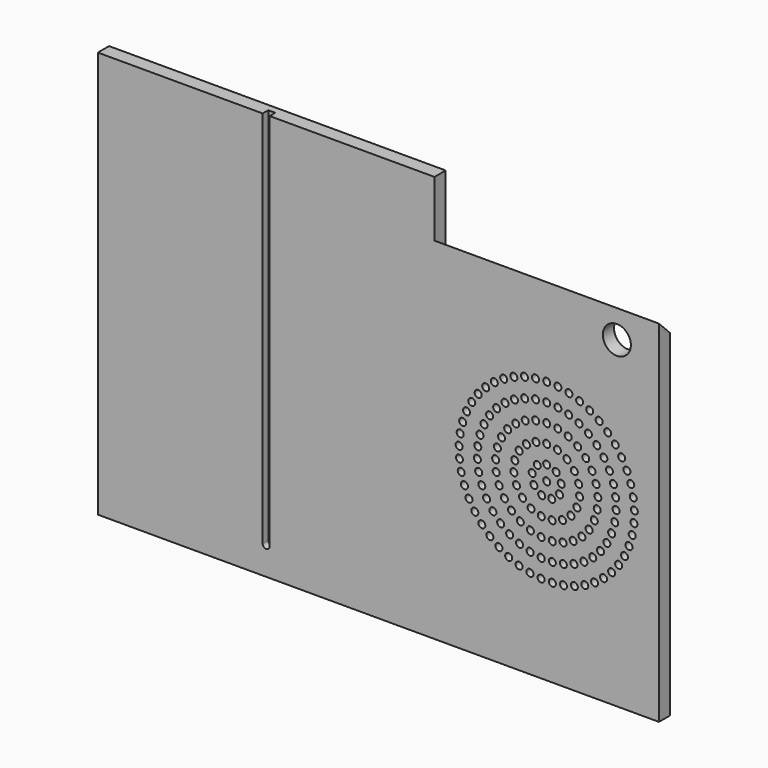
from build123d import *

# Parameters (mm, degrees)
F0_W     = 80
F0_H     = 125
F0_R     = 35
F0_R_2   = 5
F0_R_3   = 1.25
F1_DEPTH = 5
F2_DEPTH = 2.5
F3_SIZE2 = 4.99999
F3_SIZE  = 4.99999


# Not quite as in the source:
# - a fillet or chamfer is up to 0.001 mm smaller than in the source, because OpenCascade refuses the exact size


with BuildPart() as f1:
    # F0 (on Front) → F1 (new body)
    with BuildSketch(Plane.XZ):
        with BuildLine():
            Line((-78.9264041185, -49.894323349), (-78.9264041185, 75.105676651))
            Line((-78.9264041185, 75.105676651), (-78.9264041185, 95.105676651))
            Line((-78.9264041185, 95.105676651), (-137.6764041185, 95.105676651))
            Line((-137.6764041185, 95.105676651), (-137.6764041185, -39.8327037927))
            ThreePointArc((-137.6764041185, -39.8327037927), (-138.8948255892, -41.1447029883), (-140.1764041185, -39.894323349))
            Line((-140.1764041185, -39.894323349), (-140.1764041185, 95.105676651))
            Line((-140.1764041185, 95.105676651), (-198.9264041185, 95.105676651))
            Line((-198.9264041185, 95.105676651), (-198.9264041185, -49.894323349))
            Line((-198.9264041185, -49.894323349), (-78.9264041185, -49.894323349))
        make_face()
        with Locations((-38.9264041185, 12.605676651)):
            Rectangle(F0_W, F0_H)
        with Locations((-38.9264041185, 12.605676651)):
            Circle(F0_R, mode=Mode.SUBTRACT)
        with Locations((-13.9264041185, 65.105676651)):
            Circle(F0_R_2, mode=Mode.SUBTRACT)
        with Locations((-38.9264041185, 12.605676651)):
            Circle(F0_R)
        with Locations((-52.485270966, -15.5496004709)):
            Circle(F0_R_3, mode=Mode.SUBTRACT)
        with Locations((-40.9285984929, -18.5801168724)):
            Circle(F0_R_3, mode=Mode.SUBTRACT)
        with Locations((-36.9242097441, -18.5801168724)):
            Circle(F0_R_3, mode=Mode.SUBTRACT)
        with Locations((-48.7735359318, -17.0523154431)):
            Circle(F0_R_3, mode=Mode.SUBTRACT)
        with Locations((-44.9001112655, -18.068047005)):
            Circle(F0_R_3, mode=Mode.SUBTRACT)
        with Locations((-32.9526969716, -18.068047005)):
            Circle(F0_R_3, mode=Mode.SUBTRACT)
        with Locations((-29.0792723053, -17.0523154431)):
            Circle(F0_R_3, mode=Mode.SUBTRACT)
        with Locations((-25.3675372711, -15.5496004709)):
            Circle(F0_R_3, mode=Mode.SUBTRACT)
        with Locations((-62.0600915271, -8.4037261697)):
            Circle(F0_R_3, mode=Mode.SUBTRACT)
        with Locations((-64.5567870747, -5.2729689778)):
            Circle(F0_R_3, mode=Mode.SUBTRACT)
        with Locations((-55.9743697814, -13.5845766269)):
            Circle(F0_R_3, mode=Mode.SUBTRACT)
        with Locations((-59.1835414719, -11.189509548)):
            Circle(F0_R_3, mode=Mode.SUBTRACT)
        with Locations((-55.33868991, -5.9199643662)):
            Circle(F0_R_3, mode=Mode.SUBTRACT)
        with Locations((-52.1544333152, -8.3127779662)):
            Circle(F0_R_3, mode=Mode.SUBTRACT)
        with Locations((-66.6326324427, -1.848644919)):
            Circle(F0_R_3, mode=Mode.SUBTRACT)
        with Locations((-68.2535423076, 1.8130187003)):
            Circle(F0_R_3, mode=Mode.SUBTRACT)
        with Locations((-62.068056125, 3.8292056967)):
            Circle(F0_R_3, mode=Mode.SUBTRACT)
        with Locations((-58.0978769238, -3.047346395)):
            Circle(F0_R_3, mode=Mode.SUBTRACT)
        with Locations((-51.4769192426, -0.6437410766)):
            Circle(F0_R_3, mode=Mode.SUBTRACT)
        with Locations((-60.3605328622, 0.230676651)):
            Circle(F0_R_3, mode=Mode.SUBTRACT)
        with Locations((-54.0317283349, 2.3640127081)):
            Circle(F0_R_3, mode=Mode.SUBTRACT)
        with Locations((-69.3929013742, 5.6518974649)):
            Circle(F0_R_3, mode=Mode.SUBTRACT)
        with Locations((-63.1762227566, 7.65504073)):
            Circle(F0_R_3, mode=Mode.SUBTRACT)
        with Locations((-70.0320013982, 9.6049570914)):
            Circle(F0_R_3, mode=Mode.SUBTRACT)
        with Locations((-63.6563318233, 11.6090946333)):
            Circle(F0_R_3, mode=Mode.SUBTRACT)
        with Locations((-55.8802292552, 5.850655316)):
            Circle(F0_R_3, mode=Mode.SUBTRACT)
        with Locations((-49.6867407067, 7.8857554113)):
            Circle(F0_R_3, mode=Mode.SUBTRACT)
        with Locations((-56.9359881549, 9.6531552139)):
            Circle(F0_R_3, mode=Mode.SUBTRACT)
        with Locations((-50.6362719114, 11.6353693417)):
            Circle(F0_R_3, mode=Mode.SUBTRACT)
        with Locations((-70.1603483748, 13.6072884501)):
            Circle(F0_R_3, mode=Mode.SUBTRACT)
        with Locations((-69.7758348502, 17.5931733708)):
            Circle(F0_R_3, mode=Mode.SUBTRACT)
        with Locations((-63.4959487525, 15.5889594873)):
            Circle(F0_R_3, mode=Mode.SUBTRACT)
        with Locations((-68.8847745259, 21.4971637332)):
            Circle(F0_R_3, mode=Mode.SUBTRACT)
        with Locations((-62.6992273814, 19.4915588829)):
            Circle(F0_R_3, mode=Mode.SUBTRACT)
        with Locations((-57.1496389213, 13.5937117327)):
            Circle(F0_R_3, mode=Mode.SUBTRACT)
        with Locations((-56.511191482, 17.4880688292)):
            Circle(F0_R_3, mode=Mode.SUBTRACT)
        with Locations((-50.3168572433, 15.4901311249)):
            Circle(F0_R_3, mode=Mode.SUBTRACT)
        with Locations((-55.0504989297, 21.1541306938)):
            Circle(F0_R_3, mode=Mode.SUBTRACT)
        with Locations((-44.8494668097, -11.4251333303)):
            Circle(F0_R_3, mode=Mode.SUBTRACT)
        with Locations((-48.6275777126, -10.1638145796)):
            Circle(F0_R_3, mode=Mode.SUBTRACT)
        with Locations((-40.9179516943, -12.0640667253)):
            Circle(F0_R_3, mode=Mode.SUBTRACT)
        with Locations((-36.9348565428, -12.0640667253)):
            Circle(F0_R_3, mode=Mode.SUBTRACT)
        with Locations((-44.7536570435, -4.6889937231)):
            Circle(F0_R_3, mode=Mode.SUBTRACT)
        with Locations((-40.8995762048, -5.5373410671)):
            Circle(F0_R_3, mode=Mode.SUBTRACT)
        with Locations((-36.9532320323, -5.5373410671)):
            Circle(F0_R_3, mode=Mode.SUBTRACT)
        with Locations((-33.0033414274, -11.4251333303)):
            Circle(F0_R_3, mode=Mode.SUBTRACT)
        with Locations((-29.2252305245, -10.1638145796)):
            Circle(F0_R_3, mode=Mode.SUBTRACT)
        with Locations((-33.0991511936, -4.6889937231)):
            Circle(F0_R_3, mode=Mode.SUBTRACT)
        with Locations((-25.6983749219, -8.3127779662)):
            Circle(F0_R_3, mode=Mode.SUBTRACT)
        with Locations((-48.335262012, -3.0319668141)):
            Circle(F0_R_3, mode=Mode.SUBTRACT)
        with Locations((-44.5187859867, 2.2718600743)):
            Circle(F0_R_3, mode=Mode.SUBTRACT)
        with Locations((-40.8603905543, 1.015931336)):
            Circle(F0_R_3, mode=Mode.SUBTRACT)
        with Locations((-36.9924176827, 1.015931336)):
            Circle(F0_R_3, mode=Mode.SUBTRACT)
        with Locations((-29.5175462251, -3.0319668141)):
            Circle(F0_R_3, mode=Mode.SUBTRACT)
        with Locations((-26.3758889945, -0.6437410766)):
            Circle(F0_R_3, mode=Mode.SUBTRACT)
        with Locations((-33.3340222504, 2.2718600743)):
            Circle(F0_R_3, mode=Mode.SUBTRACT)
        with Locations((-21.8784384557, -13.5845766269)):
            Circle(F0_R_3, mode=Mode.SUBTRACT)
        with Locations((-18.6692667652, -11.189509548)):
            Circle(F0_R_3, mode=Mode.SUBTRACT)
        with Locations((-22.5141183271, -5.9199643662)):
            Circle(F0_R_3, mode=Mode.SUBTRACT)
        with Locations((-15.7927167099, -8.4037261697)):
            Circle(F0_R_3, mode=Mode.SUBTRACT)
        with Locations((-13.2960211624, -5.2729689778)):
            Circle(F0_R_3, mode=Mode.SUBTRACT)
        with Locations((-19.7549313133, -3.047346395)):
            Circle(F0_R_3, mode=Mode.SUBTRACT)
        with Locations((-23.8210799022, 2.3640127081)):
            Circle(F0_R_3, mode=Mode.SUBTRACT)
        with Locations((-17.4922753749, 0.230676651)):
            Circle(F0_R_3, mode=Mode.SUBTRACT)
        with Locations((-15.7847521121, 3.8292056967)):
            Circle(F0_R_3, mode=Mode.SUBTRACT)
        with Locations((-11.2201757944, -1.848644919)):
            Circle(F0_R_3, mode=Mode.SUBTRACT)
        with Locations((-9.5992659295, 1.8130187003)):
            Circle(F0_R_3, mode=Mode.SUBTRACT)
        with Locations((-47.5711600689, 4.6476181844)):
            Circle(F0_R_3, mode=Mode.SUBTRACT)
        with Locations((-40.722009871, 7.6722903919)):
            Circle(F0_R_3, mode=Mode.SUBTRACT)
        with Locations((-37.1307983661, 7.6722903919)):
            Circle(F0_R_3, mode=Mode.SUBTRACT)
        with Locations((-43.4730374884, 9.980676651)):
            Circle(F0_R_3, mode=Mode.SUBTRACT)
        with Locations((-44.0966448219, 13.5173295838)):
            Circle(F0_R_3, mode=Mode.SUBTRACT)
        with Locations((-38.9264041185, 12.605676651)):
            Circle(F0_R_3, mode=Mode.SUBTRACT)
        with Locations((-30.2816481681, 4.6476181844)):
            Circle(F0_R_3, mode=Mode.SUBTRACT)
        with Locations((-28.1660675303, 7.8857554113)):
            Circle(F0_R_3, mode=Mode.SUBTRACT)
        with Locations((-34.3797707487, 9.980676651)):
            Circle(F0_R_3, mode=Mode.SUBTRACT)
        with Locations((-33.7561634152, 13.5173295838)):
            Circle(F0_R_3, mode=Mode.SUBTRACT)
        with Locations((-27.2165363257, 11.6353693417)):
            Circle(F0_R_3, mode=Mode.SUBTRACT)
        with Locations((-42.3010390694, 16.6274099774)):
            Circle(F0_R_3, mode=Mode.SUBTRACT)
        with Locations((-38.9264041185, 17.855676651)):
            Circle(F0_R_3, mode=Mode.SUBTRACT)
        with Locations((-48.7631102381, 19.0323175089)):
            Circle(F0_R_3, mode=Mode.SUBTRACT)
        with Locations((-46.1434034926, 21.8780776364)):
            Circle(F0_R_3, mode=Mode.SUBTRACT)
        with Locations((-35.5517691677, 16.6274099774)):
            Circle(F0_R_3, mode=Mode.SUBTRACT)
        with Locations((-27.5359509938, 15.4901311249)):
            Circle(F0_R_3, mode=Mode.SUBTRACT)
        with Locations((-31.7094047444, 21.8780776364)):
            Circle(F0_R_3, mode=Mode.SUBTRACT)
        with Locations((-29.089697999, 19.0323175089)):
            Circle(F0_R_3, mode=Mode.SUBTRACT)
        with Locations((-21.9725789819, 5.850655316)):
            Circle(F0_R_3, mode=Mode.SUBTRACT)
        with Locations((-14.6765854805, 7.65504073)):
            Circle(F0_R_3, mode=Mode.SUBTRACT)
        with Locations((-20.9168200822, 9.6531552139)):
            Circle(F0_R_3, mode=Mode.SUBTRACT)
        with Locations((-14.1964764138, 11.6090946333)):
            Circle(F0_R_3, mode=Mode.SUBTRACT)
        with Locations((-8.4599068629, 5.6518974649)):
            Circle(F0_R_3, mode=Mode.SUBTRACT)
        with Locations((-7.8208068389, 9.6049570914)):
            Circle(F0_R_3, mode=Mode.SUBTRACT)
        with Locations((-20.7031693158, 13.5937117327)):
            Circle(F0_R_3, mode=Mode.SUBTRACT)
        with Locations((-21.3416167551, 17.4880688292)):
            Circle(F0_R_3, mode=Mode.SUBTRACT)
        with Locations((-14.3568594846, 15.5889594873)):
            Circle(F0_R_3, mode=Mode.SUBTRACT)
        with Locations((-22.8023093074, 21.1541306938)):
            Circle(F0_R_3, mode=Mode.SUBTRACT)
        with Locations((-15.1535808557, 19.4915588829)):
            Circle(F0_R_3, mode=Mode.SUBTRACT)
        with Locations((-7.6924598623, 13.6072884501)):
            Circle(F0_R_3, mode=Mode.SUBTRACT)
        with Locations((-8.0769733868, 17.5931733708)):
            Circle(F0_R_3, mode=Mode.SUBTRACT)
        with Locations((-8.9680337111, 21.4971637332)):
            Circle(F0_R_3, mode=Mode.SUBTRACT)
        with Locations((-67.5017985878, 25.2551561236)):
            Circle(F0_R_3, mode=Mode.SUBTRACT)
        with Locations((-65.6496154625, 28.8054444107)):
            Circle(F0_R_3, mode=Mode.SUBTRACT)
        with Locations((-61.2868023751, 23.2158175457)):
            Circle(F0_R_3, mode=Mode.SUBTRACT)
        with Locations((-59.2952547994, 26.6652791326)):
            Circle(F0_R_3, mode=Mode.SUBTRACT)
        with Locations((-52.8358616246, 24.4204763483)):
            Circle(F0_R_3, mode=Mode.SUBTRACT)
        with Locations((-49.9708335458, 27.1343751001)):
            Circle(F0_R_3, mode=Mode.SUBTRACT)
        with Locations((-56.7761646903, 29.7506044004)):
            Circle(F0_R_3, mode=Mode.SUBTRACT)
        with Locations((-63.3586379457, 32.0897329591)):
            Circle(F0_R_3, mode=Mode.SUBTRACT)
        with Locations((-60.6664838249, 35.0540938416)):
            Circle(F0_R_3, mode=Mode.SUBTRACT)
        with Locations((-53.7947751584, 32.3918850452)):
            Circle(F0_R_3, mode=Mode.SUBTRACT)
        with Locations((-50.4283026266, 34.5207132859)):
            Circle(F0_R_3, mode=Mode.SUBTRACT)
        with Locations((-57.6173581964, 37.6498523344)):
            Circle(F0_R_3, mode=Mode.SUBTRACT)
        with Locations((-54.2613276187, 39.8343861549)):
            Circle(F0_R_3, mode=Mode.SUBTRACT)
        with Locations((-50.653498021, 41.5718253181)):
            Circle(F0_R_3, mode=Mode.SUBTRACT)
        with Locations((-42.7416228817, 23.719029241)):
            Circle(F0_R_3, mode=Mode.SUBTRACT)
        with Locations((-38.9264041185, 24.355676651)):
            Circle(F0_R_3, mode=Mode.SUBTRACT)
        with Locations((-46.589380222, 29.16892806)):
            Circle(F0_R_3, mode=Mode.SUBTRACT)
        with Locations((-42.8496146524, 30.4290017927)):
            Circle(F0_R_3, mode=Mode.SUBTRACT)
        with Locations((-38.9264041185, 30.855676651)):
            Circle(F0_R_3, mode=Mode.SUBTRACT)
        with Locations((-35.1111853554, 23.719029241)):
            Circle(F0_R_3, mode=Mode.SUBTRACT)
        with Locations((-25.0169466125, 24.4204763483)):
            Circle(F0_R_3, mode=Mode.SUBTRACT)
        with Locations((-27.8819746913, 27.1343751001)):
            Circle(F0_R_3, mode=Mode.SUBTRACT)
        with Locations((-31.2634280151, 29.16892806)):
            Circle(F0_R_3, mode=Mode.SUBTRACT)
        with Locations((-35.0031935847, 30.4290017927)):
            Circle(F0_R_3, mode=Mode.SUBTRACT)
        with Locations((-46.7639369651, 36.0819535892)):
            Circle(F0_R_3, mode=Mode.SUBTRACT)
        with Locations((-42.8965833198, 37.0351706513)):
            Circle(F0_R_3, mode=Mode.SUBTRACT)
        with Locations((-38.9264041185, 37.355676651)):
            Circle(F0_R_3, mode=Mode.SUBTRACT)
        with Locations((-31.088871272, 36.0819535892)):
            Circle(F0_R_3, mode=Mode.SUBTRACT)
        with Locations((-24.0580330786, 32.3918850452)):
            Circle(F0_R_3, mode=Mode.SUBTRACT)
        with Locations((-27.4245056105, 34.5207132859)):
            Circle(F0_R_3, mode=Mode.SUBTRACT)
        with Locations((-34.9562249173, 37.0351706513)):
            Circle(F0_R_3, mode=Mode.SUBTRACT)
        with Locations((-18.5575534377, 26.6652791326)):
            Circle(F0_R_3, mode=Mode.SUBTRACT)
        with Locations((-16.5660058619, 23.2158175457)):
            Circle(F0_R_3, mode=Mode.SUBTRACT)
        with Locations((-21.0766435468, 29.7506044004)):
            Circle(F0_R_3, mode=Mode.SUBTRACT)
        with Locations((-12.2031927746, 28.8054444107)):
            Circle(F0_R_3, mode=Mode.SUBTRACT)
        with Locations((-10.3510096493, 25.2551561236)):
            Circle(F0_R_3, mode=Mode.SUBTRACT)
        with Locations((-14.4941702914, 32.0897329591)):
            Circle(F0_R_3, mode=Mode.SUBTRACT)
        with Locations((-17.1863244122, 35.0540938416)):
            Circle(F0_R_3, mode=Mode.SUBTRACT)
        with Locations((-20.2354500407, 37.6498523344)):
            Circle(F0_R_3, mode=Mode.SUBTRACT)
        with Locations((-23.5914806184, 39.8343861549)):
            Circle(F0_R_3, mode=Mode.SUBTRACT)
        with Locations((-46.8531098657, 42.833641121)):
            Circle(F0_R_3, mode=Mode.SUBTRACT)
        with Locations((-42.9225654212, 43.599114583)):
            Circle(F0_R_3, mode=Mode.SUBTRACT)
        with Locations((-38.9264041185, 43.855676651)):
            Circle(F0_R_3, mode=Mode.SUBTRACT)
        with Locations((-30.9996983714, 42.833641121)):
            Circle(F0_R_3, mode=Mode.SUBTRACT)
        with Locations((-34.9302428159, 43.599114583)):
            Circle(F0_R_3, mode=Mode.SUBTRACT)
        with Locations((-27.1993102161, 41.5718253181)):
            Circle(F0_R_3, mode=Mode.SUBTRACT)
    extrude(amount=F1_DEPTH)

    # F0 (on Front) → F2 (join)
    with BuildSketch(Plane.XZ):
        with BuildLine():
            Line((-137.6764041185, -39.8327037927), (-137.6764041185, 95.105676651))
            Line((-137.6764041185, 95.105676651), (-140.1764041185, 95.105676651))
            Line((-140.1764041185, 95.105676651), (-140.1764041185, -39.894323349))
            ThreePointArc((-140.1764041185, -39.894323349), (-138.8948255892, -41.1447029883), (-137.6764041185, -39.8327037927))
        make_face()
    extrude(amount=F2_DEPTH)

    # F3 (size 5 and 5 in the source; OpenCascade refuses exactly that, so slightly less here)
    f3_edges = [f1.edges().sort_by_distance(p)[0] for p in [
        (-38.926404, 0, 75.105677),
    ]]
    chamfer(f3_edges, length=F3_SIZE, length2=F3_SIZE2)


solid = f1.part
